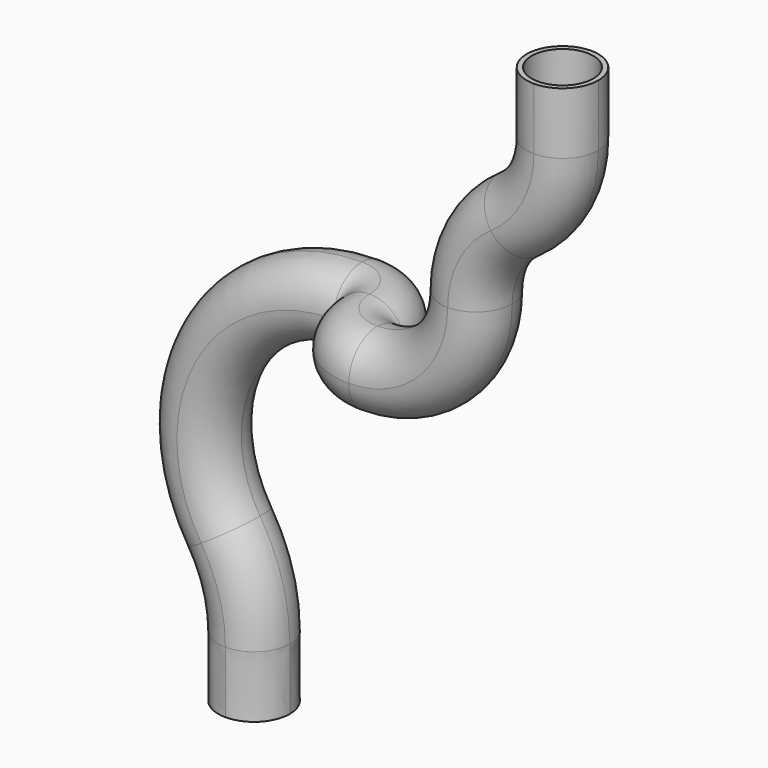
from build123d import *

# Parameters (mm, degrees)
F0_W     = 3.683
F0_H     = 3.683
F0_R     = 1.5875
F7_R     = 1.84149
F8_DEPTH = 3.175


# Not quite as in the source:
# - a fillet or chamfer is up to 0.001 mm smaller than in the source, because OpenCascade refuses the exact size


with BuildPart() as f6:
    # F6: sweep along a path in F1, F3, F5
    with BuildLine(Plane.XZ) as f6_path:
        ThreePointArc((0, 0), (-0.3184817979, 2.2424318268), (-1.2487386917, 4.3075113083))
        ThreePointArc((-1.2487386917, 4.3075113083), (-1.4990333587, 12.4990284732), (5.55625, 16.66875))
    with BuildLine(Plane.XY.offset(16.66875)) as f6_path_2:
        ThreePointArc((5.55625, 0), (6.9594150189, -0.5812099811), (7.540625, -1.984375))
        ThreePointArc((7.540625, -1.984375), (8.1218349811, -3.3875400189), (9.525, -3.96875))
    with BuildLine(Plane.XZ.offset(3.96875)) as f6_path_3:
        ThreePointArc((9.525, 16.66875), (13.1240397855, 18.1595210907), (14.6148108762, 21.7585608762))
        ThreePointArc((14.6148108762, 21.7585608762), (15.2032212708, 24.1341804711), (16.8324054381, 25.9605304381))
        ThreePointArc((16.8324054381, 25.9605304381), (18.4615896054, 27.786880405), (19.05, 30.1625))
        Line((19.05, 30.1625), (19.05, 33.3375))
    # F0 (on Top) → F6 (sweep)
    with BuildSketch(Plane.XY):
        Rectangle(F0_W, F0_H)
        Circle(F0_R, mode=Mode.SUBTRACT)
    sweep(path=f6_path.line + f6_path_2.line + f6_path_3.line)

    # F7 (radius 1.8415 in the source; OpenCascade refuses exactly that, so slightly less here)
    f7_edges = [f6.edges().sort_by_distance(p)[0] for p in [
        (1.450197, 1.8415, 2.755168),
        (-2.08716, 1.8415, 1.729696),
        (-3.112237, 1.8415, 13.387114),
        (-3.112237, -1.8415, 13.387114),
        (-2.08716, -1.8415, 1.729696),
        (1.450197, -1.8415, 2.755168),
        (0.114171, -1.8415, 11.610943),
        (0.114171, 1.8415, 11.610943),
        (8.261552, 0.720927, 18.51025),
        (9.423972, -2.085403, 18.51025),
        (11.821903, -2.12725, 19.461658),
        (13.574609, -2.12725, 24.993683),
        (16.832977, -2.12725, 28.646383),
        (17.2085, -2.12725, 31.75),
        (8.261552, 0.720927, 14.82725),
        (9.423972, -2.085403, 14.82725),
        (14.426177, -2.12725, 16.857384),
        (16.831834, -2.12725, 23.274678),
        (20.090202, -2.12725, 26.927378),
        (20.8915, -2.12725, 31.75),
        (5.657278, -1.883347, 18.51025),
        (6.819698, -4.689677, 18.51025),
        (11.821903, -5.81025, 19.461658),
        (13.574609, -5.81025, 24.993683),
        (16.832977, -5.81025, 28.646383),
        (17.2085, -5.81025, 31.75),
        (5.657278, -1.883347, 14.82725),
        (6.819698, -4.689677, 14.82725),
        (14.426177, -5.81025, 16.857384),
        (16.831834, -5.81025, 23.274678),
        (20.090202, -5.81025, 26.927378),
        (20.8915, -5.81025, 31.75),
    ]]
    fillet(f7_edges, radius=F7_R)

    # F8 (add): a face of the model
    f8_faces = [f6.faces().sort_by_distance(p)[0] for p in [
        (1.7894145117, 0, 0),
    ]]
    extrude(f8_faces, amount=F8_DEPTH)


solid = f6.part
